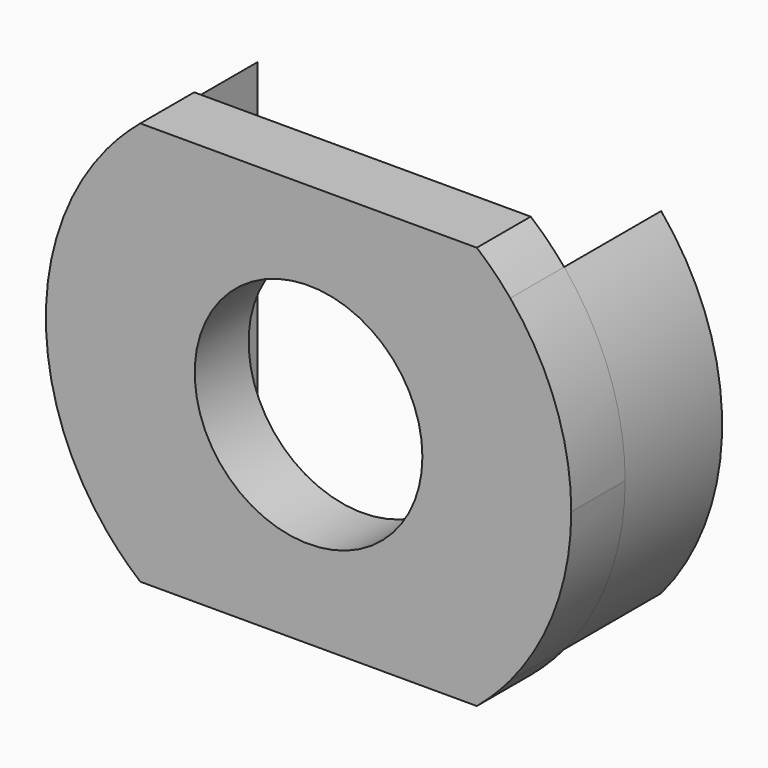
from build123d import *

# Parameters (mm, degrees)
F0_R     = 8.45
F1_DEPTH = 5
F3_DEPTH = 5
F5_DEPTH = 9


# Not quite as in the source:
# - after a boolean that leaves OpenCascade's solid faulty, fix() repairs it
# - a feature names something its author has since deleted; it is built from what else it names


with BuildPart() as f1:
    # F0 (on Front) → F1 (new body)
    with BuildSketch(Plane.XZ):
        with BuildLine():
            ThreePointArc((14.975, 12.4899709767), (13.7885822331, 13.7885822331), (12.4899709767, 14.975))
            Line((12.4899709767, 14.975), (-12.4899709767, 14.975))
            ThreePointArc((-12.4899709767, 14.975), (-13.7885822331, 13.7885822331), (-14.975, 12.4899709767))
            Line((-14.975, 12.4899709767), (-14.975, -12.4899709767))
            ThreePointArc((-14.975, -12.4899709767), (-13.7885822331, -13.7885822331), (-12.4899709767, -14.975))
            Line((-12.4899709767, -14.975), (12.4899709767, -14.975))
            ThreePointArc((12.4899709767, -14.975), (13.7885822331, -13.7885822331), (14.975, -12.4899709767))
            Line((14.975, -12.4899709767), (14.975, 12.4899709767))
        make_face()
        Circle(F0_R, mode=Mode.SUBTRACT)
        with BuildLine():
            Line((-12.4899709767, 14.975), (12.4899709767, 14.975))
            ThreePointArc((12.4899709767, 14.975), (0, 19.5), (-12.4899709767, 14.975))
        make_face()
        with BuildLine():
            ThreePointArc((-12.4899709767, -14.975), (0, -19.5), (12.4899709767, -14.975))
            Line((12.4899709767, -14.975), (-12.4899709767, -14.975))
        make_face()
        with BuildLine():
            ThreePointArc((19.5, 0), (18.3338825675, 6.6421946674), (14.975, 12.4899709767))
            Line((14.975, 12.4899709767), (14.975, -12.4899709767))
            ThreePointArc((14.975, -12.4899709767), (18.3338825675, -6.6421946674), (19.5, 0))
        make_face()
        with BuildLine():
            Line((-14.975, -12.4899709767), (-14.975, 12.4899709767))
            ThreePointArc((-14.975, 12.4899709767), (-19.5, 0), (-14.975, -12.4899709767))
        make_face()
    extrude(amount=F1_DEPTH)

    # F2 (on face) → F3 (cut, through all)
    with BuildSketch(Plane(origin=(0, 0, 0), x_dir=(-1, 0, 0), z_dir=(0, 1, 0))):
        with BuildLine():
            ThreePointArc((12.4899709767, 14.975), (0, 19.5), (-12.4899709767, 14.975))
            Line((-12.4899709767, 14.975), (12.4899709767, 14.975))
        make_face()
        with BuildLine():
            Line((12.4899709767, -14.975), (-12.4899709767, -14.975))
            ThreePointArc((-12.4899709767, -14.975), (0, -19.5), (12.4899709767, -14.975))
        make_face()
    extrude(amount=-F3_DEPTH, mode=Mode.SUBTRACT)

    # F4 (on face) → F5 (join)
    with BuildSketch(Plane(origin=(0, 0, 0), x_dir=(-1, 0, 0), z_dir=(0, 1, 0))):
        with BuildLine():
            Line((-14.975, -12.4899709767), (-14.975, 12.4899709767))
            ThreePointArc((-14.975, 12.4899709767), (-19.5, 0), (-14.975, -12.4899709767))
        make_face()
        with BuildLine():
            ThreePointArc((14.975, -12.4899709767), (19.5, 0), (14.975, 12.4899709767))
            Line((14.975, 12.4899709767), (14.975, -12.4899709767))
        make_face()
    extrude(amount=F5_DEPTH)

    add(f1.part.fix(), mode=Mode.REPLACE)


solid = f1.part
